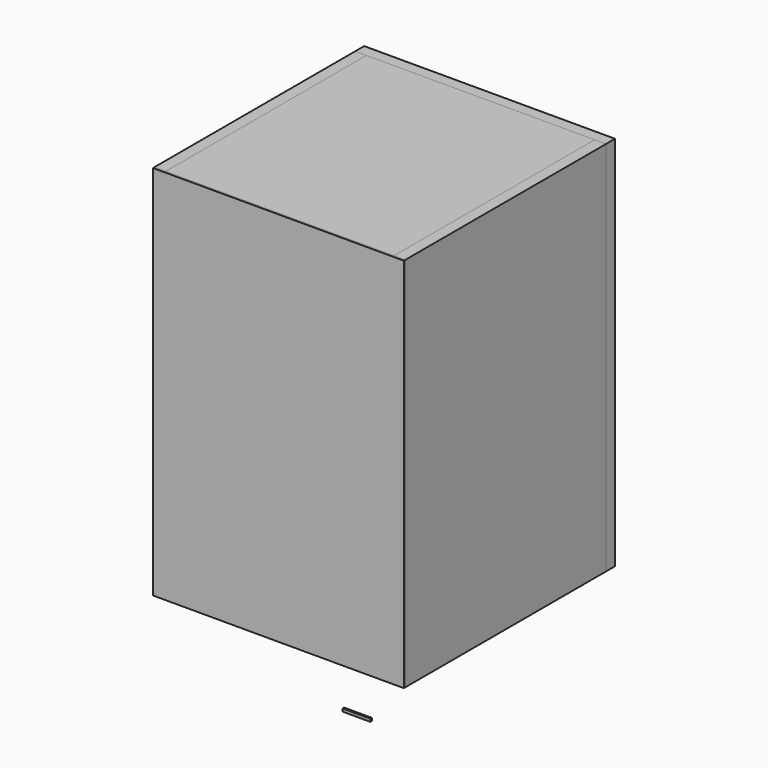
from build123d import *

# Parameters (mm, degrees)
F0_W      = 2000
F0_H      = 3000
F1_DEPTH  = 15
F0_W_2    = 223.0252540781
F0_H_2    = 22.3025142319
F2_W      = 90
F2_H      = 3000
F3_DEPTH  = 2000
F5_DEPTH  = 120
F7_DEPTH  = 1820
F8_W      = 234.393119812
F8_H      = 71.7555948407
F9_DEPTH  = 50
F11_DEPTH = 1820
F12_W     = 2000
F12_H     = 90
F12_W_2   = 0.0563644571
F13_DEPTH = 1820
F14_W     = 2000
F14_H     = 3000
F15_DEPTH = 90
F16_W     = 2000
F16_H     = 3000
F17_DEPTH = 90
F18_R     = 350.2358859711
F19_DEPTH = 90


# Not quite as in the source:
# - ends of sketch curves that miss each other by under 0.0002 mm in the source are joined


with BuildPart() as f1:
    # F0 (on Front) → F1 (new body)
    with BuildSketch(Plane.XZ):
        with Locations((1000, 1500)):
            Rectangle(F0_W, F0_H)
    extrude(amount=F1_DEPTH)


with BuildPart() as f1b:
    # F0 (on Front) → F1, piece 2 (new body)
    with BuildSketch(Plane.XZ):
        with Locations((1622.508082666, -312.2352271864)):
            Rectangle(F0_W_2, F0_H_2)
    extrude(amount=F1_DEPTH)


with BuildPart() as f3:
    # F2 (on face) → F3 (new body)
    with BuildSketch(Plane(origin=(0, 0, 0), x_dir=(-1, 0, 0), z_dir=(0, 1, 0))):
        with Locations((-45, 1500)):
            Rectangle(F2_W, F2_H)
    extrude(amount=F3_DEPTH)


with BuildPart() as f5:
    # F4 (on face) → F5 (new body)
    with BuildSketch(Plane.YZ.offset(90)):
        Polygon((169.0563857555, 1070.8147287369), (0, 1253.195643425), (0, 906.6718220711), align=None)
    extrude(amount=F5_DEPTH)


with BuildPart() as f7:
    # F6 (on face) → F7 (new body)
    with BuildSketch(Plane.YZ.offset(90)):
        Polygon((0, 1253.1963586807), (169.0228581429, 1070.8320140839), (219.0007353757, 1117.1535890194), (49.9778772329, 1299.5179336163), align=None)
    extrude(amount=F7_DEPTH)


with BuildPart() as f9:
    # F8 (on face) → F9 (new body)
    with BuildSketch(Plane(origin=(0, 674.7720834381, 625.4068271396), x_dir=(-1, 0, 0), z_dir=(0, 0.733425793, 0.6797695243))):
        with Locations((-916.9374704361, 706.3570286676)):
            Rectangle(F8_W, F8_H)
    extrude(amount=F9_DEPTH)


with BuildPart() as f11:
    # F10 (on face) → F11 (new body)
    with BuildSketch(Plane.YZ.offset(90)):
        Polygon((2000, 2910), (2000, 3000), (0, 3000), (0, 2910), (434.6059262753, 2910), (667.1281456947, 2910), align=None)
    extrude(amount=F11_DEPTH)


with BuildPart() as f13:
    # F12 (on face) → F13 (new body)
    with BuildSketch(Plane.YZ.offset(90)):
        with Locations((1000, 45)):
            Rectangle(F12_W, F12_H)
        with Locations((-0.0281822286, 45)):
            Rectangle(F12_W_2, F12_H)
        Polygon((-0.0563644571, 90), (0, 90), (0, 111.4134863019), (-0.0564195216, 111.4134863019), align=None)
    extrude(amount=F13_DEPTH)


with BuildPart() as f15:
    # F14 (on face) → F15 (new body)
    with BuildSketch(Plane.YZ.offset(1910)):
        with Locations((1000, 1500)):
            Rectangle(F14_W, F14_H)
    extrude(amount=F15_DEPTH)


with BuildPart() as f17:
    # F16 (on face) → F17 (new body)
    with BuildSketch(Plane(origin=(0, 2000, 0), x_dir=(-1, 0, 0), z_dir=(0, 1, 0))):
        with Locations((-1000, 1500)):
            Rectangle(F16_W, F16_H)
    extrude(amount=F17_DEPTH)

    # F18 (on face) → F19 (cut)
    with BuildSketch(Plane(origin=(0, 2090, 0), x_dir=(-1, 0, 0), z_dir=(0, 1, 0))):
        with Locations((-1225.5524396896, 678.6203980446)):
            Circle(F18_R)
    extrude(amount=-F19_DEPTH, mode=Mode.SUBTRACT)


solid = Compound([f1.part, f1b.part, f3.part, f5.part, f7.part, f9.part, f11.part, f13.part, f15.part, f17.part])
